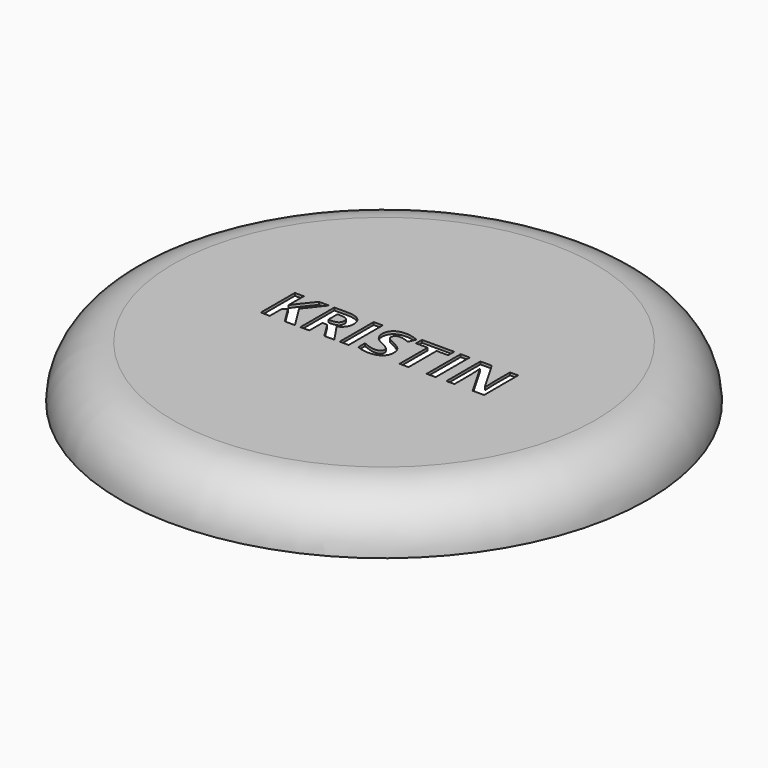
from build123d import *

# Parameters (mm, degrees)
F0_R         = 63.5
F1_DEPTH     = 12.7
F2_R         = 12.69999
F3_SCALE     = 0.95
F5_TEXT_SIZE = 14.3274380308
F6_DEPTH     = 12.7


# Not quite as in the source:
# - a fillet or chamfer is up to 0.001 mm smaller than in the source, because OpenCascade refuses the exact size
# - Text() gives the source's letters only with a copy of the font that has no kerning and outlines rounded to 1/6400 em; it was checked with that copy


with BuildPart() as f1:
    # F0 (on Top) → F1 (new body)
    with BuildSketch(Plane.XY):
        Circle(F0_R)
    extrude(amount=F1_DEPTH)

    # F2 (radius 12.7 in the source; OpenCascade refuses exactly that, so slightly less here)
    f2_edges = [f1.edges().sort_by_distance(p)[0] for p in [
        (-63.5, 0, 12.7),
    ]]
    fillet(f2_edges, radius=F2_R)


with BuildPart() as f3_1:
    # F3: copy of F1
    add(f1.part.scale(F3_SCALE))


with BuildPart() as f1_1:
    add(f1.part)

    # F4: cut F3_1
    add(f3_1.part, mode=Mode.SUBTRACT)

    # F5 (on face) → F6 (cut)
    with BuildSketch(Plane.XY.offset(12.7)):
        with Locations((-26.9216094166, -5.0320760347)):
            Text('KRISTIN', F5_TEXT_SIZE, font='Open Sans', font_style=FontStyle.BOLD, text_align=(TextAlign.LEFT, TextAlign.BOTTOM))
    extrude(amount=-F6_DEPTH, mode=Mode.SUBTRACT)


solid = f1_1.part
